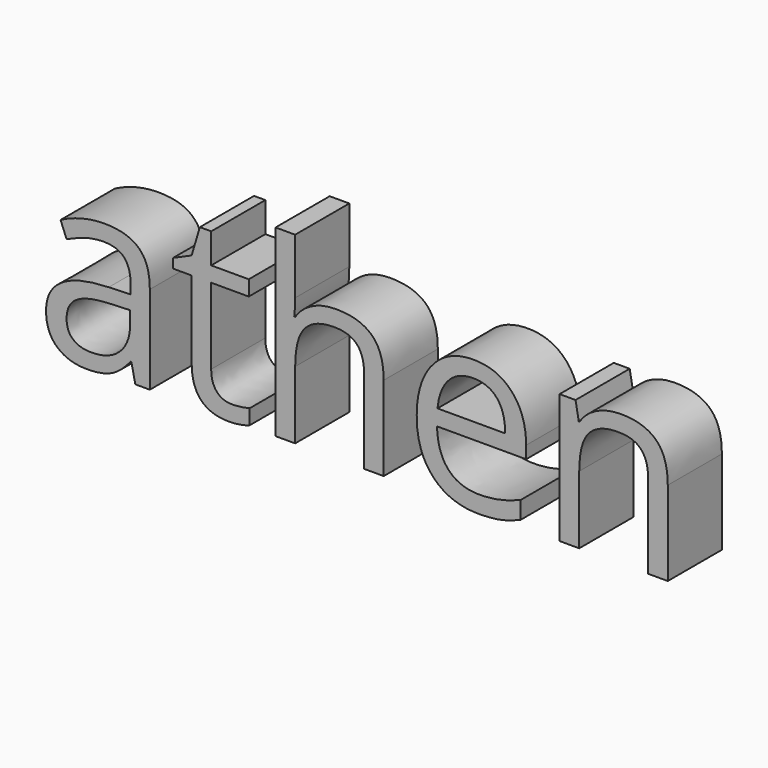
from build123d import *

# Parameters (mm, degrees)
F0_TEXT_SIZE = 107.382866554
F1_DEPTH     = 30.0586


# Not quite as in the source:
# - Text() gives the source's letters only with a copy of the font that has no kerning and outlines rounded to 1/6400 em; it was checked with that copy


with BuildPart() as f1:
    # F0 (on Front) → F1 (new body)
    with BuildSketch(Plane.XZ):
        with Locations((-18.2746127248, -48.3808610588)):
            Text('athen', F0_TEXT_SIZE, font='Open Sans', text_align=(TextAlign.LEFT, TextAlign.BOTTOM))
    extrude(amount=F1_DEPTH)


solid = f1.part
